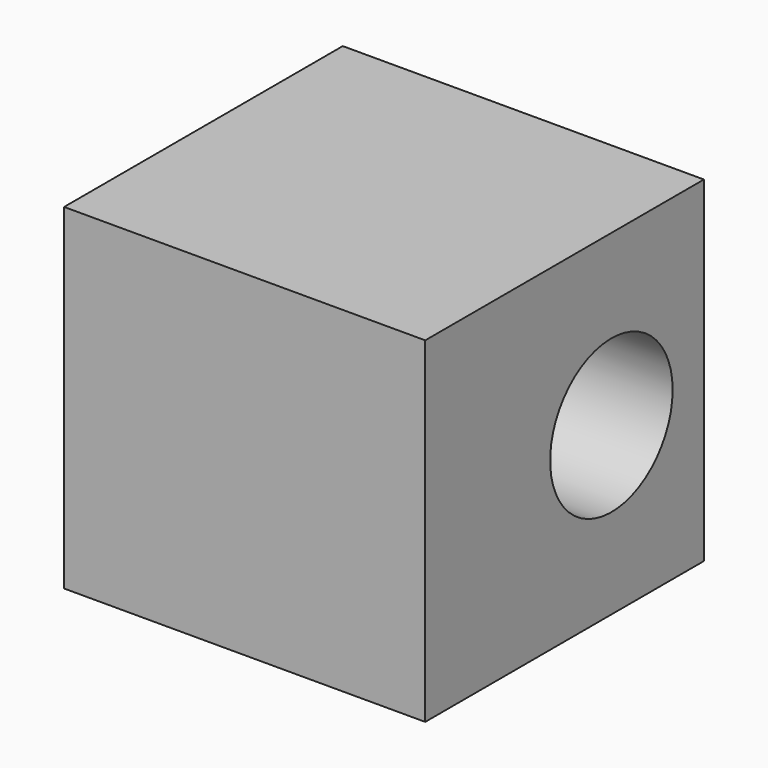
from build123d import *

# Parameters (mm, degrees)
F0_W     = 113.6151142418
F0_H     = 109.588842839
F1_DEPTH = 105.6814342737
F2_R     = 24.0827135545
F3_DEPTH = 200


# Not quite as in the source:
# - the program builds the solid bodies; features that only make, move or delete a surface that nothing else refers to are left out


with BuildPart() as f1:
    # F0 (on Top) → F1 (new body)
    with BuildSketch(Plane.XY):
        with Locations((-3.817750141, 19.6385178715)):
            Rectangle(F0_W, F0_H)
    extrude(amount=F1_DEPTH)

    # F2 (on face) → F3 (cut)
    with BuildSketch(Plane.YZ.offset(52.9898069799)):
        with Locations((38.0479171872, 52.4106435478)):
            Circle(F2_R)
    extrude(amount=-F3_DEPTH, mode=Mode.SUBTRACT)


solid = f1.part
